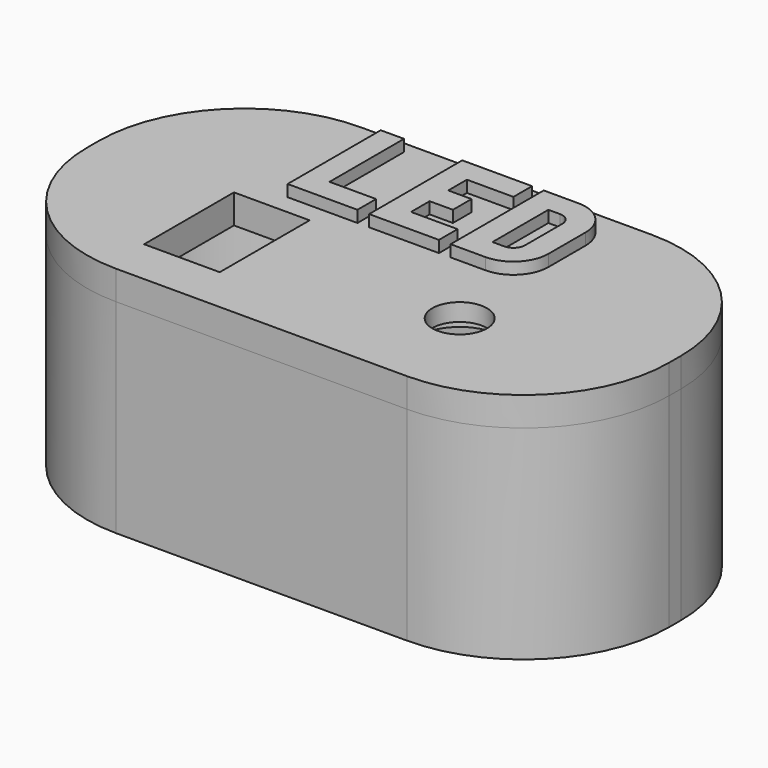
from build123d import *

# Parameters (mm, degrees)
F2_DEPTH  = 5
F3_W      = 13
F3_H      = 19.3
F3_R      = 4.7
F4_DEPTH  = 5
F5_R      = 7.1
F6_DEPTH  = 2
F8_DEPTH  = 35
F10_DEPTH = 5
F12_DEPTH = 8.75
F14_DEPTH = 2


with BuildPart() as f2:
    # F1 (on offset) → F2 (new body)
    with BuildSketch(Plane.XY.offset(35)):
        with BuildLine():
            ThreePointArc((50, 1.3), (42.6776695297, 18.9776695297), (25, 26.3))
            Line((25, 26.3), (-25, 26.3))
            ThreePointArc((-25, 26.3), (-42.6776695297, 18.9776695297), (-50, 1.3))
            Line((-50, 1.3), (-50, -1.3))
            ThreePointArc((-50, -1.3), (-42.6776695297, -18.9776695297), (-25, -26.3))
            Line((-25, -26.3), (25, -26.3))
            ThreePointArc((25, -26.3), (42.6776695297, -18.9776695297), (50, -1.3))
            Line((50, -1.3), (50, 1.3))
        make_face()
    extrude(amount=F2_DEPTH)

    # F3 (on face) → F4 (cut, through all)
    with BuildSketch(Plane.XY.offset(40)):
        with Locations((-20, -8.75)):
            Rectangle(F3_W, F3_H)
        with Locations((20, -8.75)):
            Circle(F3_R)
    extrude(amount=-F4_DEPTH, mode=Mode.SUBTRACT)

    # F5 (on face) → F6 (cut)
    with BuildSketch(Plane.XY.offset(35)):
        with Locations((20, -8.75)):
            Circle(F5_R)
    extrude(amount=F6_DEPTH, mode=Mode.SUBTRACT)


with BuildPart() as f8:
    # F7 (on face) → F8 (new body)
    with BuildSketch(Plane.XY.offset(35)):
        with BuildLine():
            ThreePointArc((50, 1.3), (42.6776695297, 18.9776695297), (25, 26.3))
            Line((25, 26.3), (-25, 26.3))
            ThreePointArc((-25, 26.3), (-42.6776695297, 18.9776695297), (-50, 1.3))
            Line((-50, 1.3), (-50, -1.3))
            ThreePointArc((-50, -1.3), (-42.6776695297, -18.9776695297), (-25, -26.3))
            Line((-25, -26.3), (25, -26.3))
            ThreePointArc((25, -26.3), (42.6776695297, -18.9776695297), (50, -1.3))
            Line((50, -1.3), (50, 1.3))
        make_face()
        with BuildLine():
            Line((-25, 21.3), (25, 21.3))
            ThreePointArc((25, 21.3), (39.1421356237, 15.4421356237), (45, 1.3))
            Line((45, 1.3), (45, -1.3))
            ThreePointArc((45, -1.3), (39.1421356237, -15.4421356237), (25, -21.3))
            Line((25, -21.3), (-25, -21.3))
            ThreePointArc((-25, -21.3), (-39.1421356237, -15.4421356237), (-45, -1.3))
            Line((-45, -1.3), (-45, 1.3))
            ThreePointArc((-45, 1.3), (-39.1421356237, 15.4421356237), (-25, 21.3))
        make_face(mode=Mode.SUBTRACT)
    extrude(amount=-F8_DEPTH)

    # F9 (on face) → F10 (cut, through all)
    with BuildSketch(Plane(origin=(0, 26.3, 0), x_dir=(-1, 0, 0), z_dir=(0, 1, 0))):
        with BuildLine():
            ThreePointArc((0, 5), (-3.5355339059, 3.5355339059), (-5, 0))
            Line((-5, 0), (5, 0))
            ThreePointArc((5, 0), (3.5355339059, 3.5355339059), (0, 5))
        make_face()
    extrude(amount=-F10_DEPTH, mode=Mode.SUBTRACT)

    # F11 (on face) → F12 (join)
    with BuildSketch(Plane.XZ.offset(-21.3)):
        Polygon((25, 35), (24.25, 35), (24.25, 8.5), (0, 8.5), (0, 7.75), (25, 7.75), align=None)
    extrude(amount=F12_DEPTH)


with BuildPart() as f14:
    # F3 (on face) → F14 (new body)
    with BuildSketch(Plane.XY.offset(40)):
        Polygon((-16, 24.3), (-20, 24.3), (-20, 4.3), (-8, 4.3), (-8, 8.3), (-16, 8.3), align=None)
    extrude(amount=F14_DEPTH)


with BuildPart() as f14b:
    # F3 (on face) → F14, piece 2 (new body)
    with BuildSketch(Plane.XY.offset(40)):
        Polygon((6, 24.3), (-6, 24.3), (-6, 4.3), (6, 4.3), (6, 8.3), (-2, 8.3), (-2, 12.3), (2, 12.3), (2, 16.3), (-2, 16.3), (-2, 20.3), (6, 20.3), align=None)
    extrude(amount=F14_DEPTH)


with BuildPart() as f14c:
    # F3 (on face) → F14, piece 3 (new body)
    with BuildSketch(Plane.XY.offset(40)):
        with BuildLine():
            Line((12, 24.3), (8, 24.3))
            Line((8, 24.3), (8, 4.3))
            Line((8, 4.3), (12, 4.3))
            Line((12, 4.3), (14, 4.3))
            ThreePointArc((14, 4.3), (18.2426406871, 6.0573593129), (20, 10.3))
            Line((20, 10.3), (20, 18.3))
            ThreePointArc((20, 18.3), (18.2426406871, 22.5426406871), (14, 24.3))
            Line((14, 24.3), (12, 24.3))
        make_face()
        with BuildLine():
            Line((12, 8.3), (12, 20.3))
            Line((12, 20.3), (14, 20.3))
            ThreePointArc((14, 20.3), (15.4142135624, 19.7142135624), (16, 18.3))
            Line((16, 18.3), (16, 10.3))
            ThreePointArc((16, 10.3), (15.4142135624, 8.8857864376), (14, 8.3))
            Line((14, 8.3), (12, 8.3))
        make_face(mode=Mode.SUBTRACT)
    extrude(amount=F14_DEPTH)


solid = Compound([f2.part, f8.part, f14.part, f14b.part, f14c.part])
